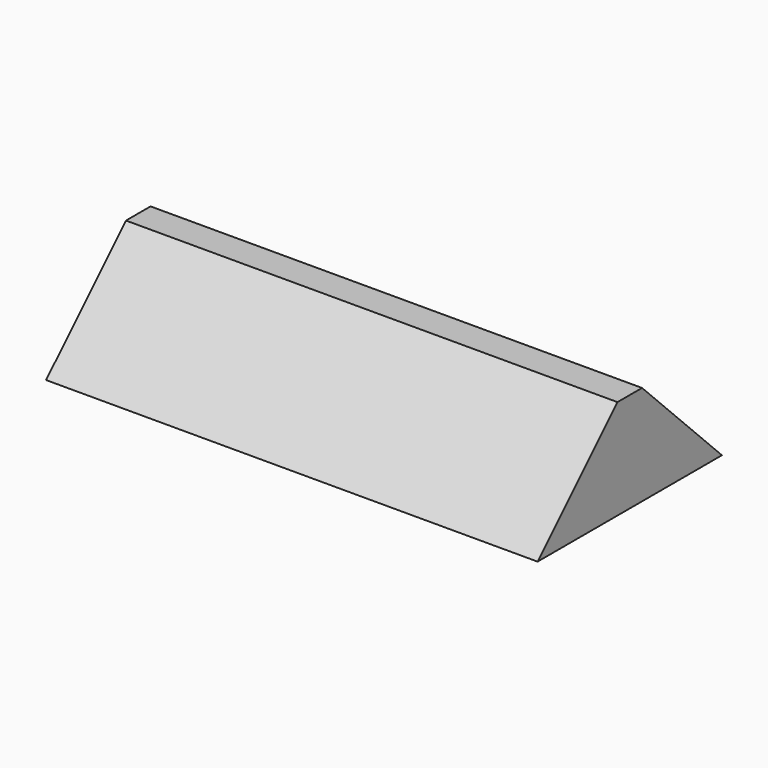
from build123d import *

# Parameters (mm, degrees)
F0_W     = 95.25
F0_H     = 41.275
F1_DEPTH = 203.2
F2_SIZE  = 41.27499


# Not quite as in the source:
# - a fillet or chamfer is up to 0.001 mm smaller than in the source, because OpenCascade refuses the exact size


with BuildPart() as f1:
    # F0 (on Right) → F1 (new body)
    with BuildSketch(Plane.YZ):
        Rectangle(F0_W, F0_H)
    extrude(amount=-F1_DEPTH)

    # F2 (size 41.275 in the source; OpenCascade refuses exactly that, so slightly less here)
    f2_edges = [f1.edges().sort_by_distance(p)[0] for p in [
        (-101.6, -47.625, 20.6375),
        (-101.6, 47.625, 20.6375),
    ]]
    chamfer(f2_edges, length=F2_SIZE)


solid = f1.part
